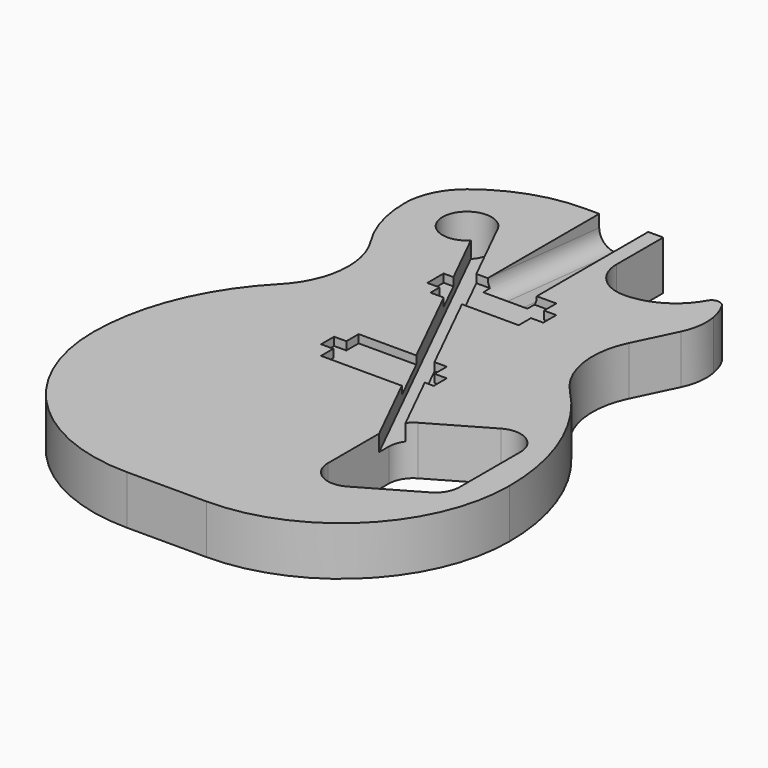
from build123d import *

# Parameters (mm, degrees)
F2_DEPTH  = 38.1
F4_R      = 19.05
F5_DEPTH  = 38.101
F11_DEPTH = 117.475
F12_W     = 9.525
F12_H     = 6.35
F13_DEPTH = 6.35
F15_DEPTH = 12.7


# Not quite as in the source:
# - a feature of the source that left no trace in its solid (it failed there, or was rolled back) is left out


with BuildPart() as f2:
    # F1 (on Top) → F2 (new body)
    with BuildSketch(Plane.XY):
        with BuildLine():
            Line((-120.142, 381.762), (0, 381.762))
            Line((0, 381.762), (0, 444.5))
            Line((0, 444.5), (-30.734, 444.5))
            ThreePointArc((-30.734, 444.5), (-68.3812374672, 438.1220807393), (-101.8270568949, 419.700096432))
            ThreePointArc((-101.8270568949, 419.700096432), (-115.3236770577, 402.8258096141), (-120.142, 381.762))
        make_face()
        with BuildLine():
            Line((0, 444.5), (0, 381.762))
            Line((0, 381.762), (36.5448035283, 381.762))
            ThreePointArc((36.5448035283, 381.762), (32.2256329717, 389.9223670283), (30.734, 399.034))
            Line((30.734, 399.034), (30.734, 444.5))
            Line((30.734, 444.5), (0, 444.5))
        make_face()
        with BuildLine():
            Line((0, 381.762), (0, 295.402))
            Line((0, 295.402), (94.869, 295.402))
            ThreePointArc((94.869, 295.402), (96.466719449, 309.5567752573), (101.1794775617, 322.9992557201))
            Line((101.1794775617, 322.9992557201), (116.4239761752, 354.5902807248))
            ThreePointArc((116.4239761752, 354.5902807248), (120.430931673, 367.882227955), (120.142, 381.762))
            Line((120.142, 381.762), (91.175550227, 381.762))
            ThreePointArc((91.175550227, 381.762), (76.2148779155, 373.3684407202), (59.309, 370.459))
            ThreePointArc((59.309, 370.459), (46.6010649789, 373.440270055), (36.5448035283, 381.762))
            Line((36.5448035283, 381.762), (0, 381.762))
        make_face()
        with BuildLine():
            ThreePointArc((103.5459630182, 396.5232874828), (98.0699350262, 388.5483304334), (91.175550227, 381.762))
            Line((91.175550227, 381.762), (120.142, 381.762))
            ThreePointArc((120.142, 381.762), (118.0226976621, 389.4849479409), (114.552023257, 396.7022733785))
            ThreePointArc((114.552023257, 396.7022733785), (112.2345927331, 398.9686730826), (109.1004928586, 399.796))
            ThreePointArc((109.1004928586, 399.796), (105.8770068198, 398.9169814255), (103.5459630182, 396.5232874828))
        make_face()
        with BuildLine():
            Line((94.869, 295.402), (0, 295.402))
            Line((0, 295.402), (0, 0))
            Line((0, 0), (30.906359714, 0))
            ThreePointArc((30.906359714, 0), (123.5505287221, 38.3744712779), (161.925, 131.018640286))
            ThreePointArc((161.925, 131.018640286), (149.2199863218, 195.80132063), (112.9871937272, 250.9864434976))
            ThreePointArc((112.9871937272, 250.9864434976), (99.5727641582, 271.4175748279), (94.869, 295.402))
        make_face()
        with BuildLine():
            Line((0, 295.402), (-94.869, 295.402))
            ThreePointArc((-94.869, 295.402), (-99.5727641582, 271.4175748279), (-112.9871937272, 250.9864434976))
            ThreePointArc((-112.9871937272, 250.9864434976), (-149.2199863218, 195.80132063), (-161.925, 131.018640286))
            ThreePointArc((-161.925, 131.018640286), (-123.5505287221, 38.3744712779), (-30.906359714, 0))
            Line((-30.906359714, 0), (0, 0))
            Line((0, 0), (0, 295.402))
        make_face()
        with BuildLine():
            ThreePointArc((-104.887559724, 329.6362744337), (-97.4250853837, 313.2370573657), (-94.869, 295.402))
            Line((-94.869, 295.402), (0, 295.402))
            Line((0, 295.402), (0, 381.762))
            Line((0, 381.762), (-120.142, 381.762))
            ThreePointArc((-120.142, 381.762), (-116.2500581541, 354.6060190108), (-104.887559724, 329.6362744337))
        make_face()
    extrude(amount=F2_DEPTH)

    # F4 (on face) → F5 (cut, through all)
    with BuildSketch(Plane.XY.offset(38.1)):
        with Locations((-71.6915, 381.762)):
            Circle(F4_R)
        with BuildLine():
            Line((139.2962010965, 110.8024764079), (139.2962010965, 170.1017752607))
            ThreePointArc((139.2962010965, 170.1017752607), (129.7712010965, 186.5995592028), (110.7212010965, 186.5995592028))
            Line((110.7212010965, 186.5995592028), (66.675, 161.169473143))
            ThreePointArc((66.675, 161.169473143), (59.7022160579, 154.1966892009), (57.15, 144.6716892009))
            Line((57.15, 144.6716892009), (57.15, 108.5037669007))
            Line((57.15, 108.5037669007), (69.5417475728, 132.0304736397))
            ThreePointArc((69.5417475728, 132.0304736397), (65.9030700587, 154.5765309479), (88.5733379566, 151.8154392009))
            Line((88.5733379566, 151.8154392009), (107.8728631399, 162.9580252607))
            ThreePointArc((107.8728631399, 162.9580252607), (116.5483239896, 183.9024405039), (134.5337010965, 170.1017752607))
            ThreePointArc((134.5337010965, 170.1017752607), (130.3489892327, 159.9989871245), (120.2462010965, 155.8142752607))
            Line((120.2462010965, 155.8142752607), (120.2462010965, 125.0899764079))
            ThreePointArc((120.2462010965, 125.0899764079), (130.3489892327, 120.9052645441), (134.5337010965, 110.8024764079))
            ThreePointArc((134.5337010965, 110.8024764079), (125.4430565732, 97.4936316269), (109.7392514861, 101.1207066247))
            Line((109.7392514861, 101.1207066247), (90.3263274862, 83.23240717))
            ThreePointArc((90.3263274862, 83.23240717), (85.8817697832, 74.8654407377), (77.1799912803, 71.1185391723))
            Line((77.1799912803, 71.1185391723), (72.3922577123, 66.7068177967))
            ThreePointArc((72.3922577123, 66.7068177967), (79.2572186381, 66.5693077763), (85.725, 68.874606406))
            Line((85.725, 68.874606406), (129.7712010965, 94.3046924658))
            ThreePointArc((129.7712010965, 94.3046924658), (136.7439850386, 101.2774764079), (139.2962010965, 110.8024764079))
        make_face()
        with BuildLine():
            Line((69.5417475728, 132.0304736397), (57.15, 108.5037669007))
            Line((57.15, 108.5037669007), (57.15, 85.3723903481))
            ThreePointArc((57.15, 85.3723903481), (61.4446621425, 73.3232200567), (72.3922577123, 66.7068177967))
            Line((72.3922577123, 66.7068177967), (77.1799912803, 71.1185391723))
            ThreePointArc((77.1799912803, 71.1185391723), (85.8817697832, 74.8654407377), (90.3263274862, 83.23240717))
            Line((90.3263274862, 83.23240717), (109.7392514861, 101.1207066247))
            ThreePointArc((109.7392514861, 101.1207066247), (125.4430565732, 97.4936316269), (134.5337010965, 110.8024764079))
            ThreePointArc((134.5337010965, 110.8024764079), (130.3489892327, 120.9052645441), (120.2462010965, 125.0899764079))
            Line((120.2462010965, 125.0899764079), (120.2462010965, 155.8142752607))
            ThreePointArc((120.2462010965, 155.8142752607), (130.3489892327, 159.9989871245), (134.5337010965, 170.1017752607))
            ThreePointArc((134.5337010965, 170.1017752607), (116.5483239896, 183.9024405039), (107.8728631399, 162.9580252607))
            Line((107.8728631399, 162.9580252607), (88.5733379566, 151.8154392009))
            ThreePointArc((88.5733379566, 151.8154392009), (65.9030700587, 154.5765309479), (69.5417475728, 132.0304736397))
        make_face()
    extrude(amount=-F5_DEPTH, mode=Mode.SUBTRACT)

    # F10 (on face) → F11 (cut)
    with BuildSketch(Plane(origin=(0, 441.123523107, -38.5933074865), x_dir=(-1, 0, 0), z_dir=(0, 0.9961946981, -0.0871557427))):
        with BuildLine():
            Line((19.05, 76.6957456486), (-19.05, 76.6957456486))
            Line((-19.05, 76.6957456486), (-19.05, 67.1707456486))
            ThreePointArc((-19.05, 67.1707456486), (-15.3302561211, 58.1904895276), (-6.35, 54.4707456486))
            Line((-6.35, 54.4707456486), (0, 54.4707456486))
            Line((0, 54.4707456486), (6.35, 54.4707456486))
            ThreePointArc((6.35, 54.4707456486), (15.3302561211, 58.1904895276), (19.05, 67.1707456486))
            Line((19.05, 67.1707456486), (19.05, 76.6957456486))
        make_face()
    extrude(amount=-F11_DEPTH, mode=Mode.SUBTRACT)

    # F12 (on face) → F13 (cut)
    with BuildSketch(Plane.XY.offset(38.1)):
        Polygon((-34.29, 299.5168), (0, 299.5168), (0, 317.8302), (-34.29, 317.8302), (-34.29, 311.4802), (-34.29, 308.3052), align=None)
        Polygon((0, 317.8302), (0, 299.5168), (34.29, 299.5168), (34.29, 311.4802), (34.29, 317.8302), align=None)
        Polygon((0, 229.6668), (-34.29, 229.6668), (-34.29, 217.7034), (-34.29, 211.3534), (0, 211.3534), align=None)
        Polygon((34.29, 229.6668), (0, 229.6668), (0, 211.3534), (34.29, 211.3534), (34.29, 217.7034), align=None)
        with Locations((-39.0525, 214.5284)):
            Rectangle(F12_W, F12_H)
        Polygon((34.29, 211.3534), (0, 211.3534), (0, 193.04), (34.29, 193.04), (34.29, 205.0034), align=None)
        Polygon((0, 193.04), (0, 211.3534), (-34.29, 211.3534), (-34.29, 205.0034), (-34.29, 193.04), align=None)
        with Locations((-39.0525, 208.1784)):
            Rectangle(F12_W, F12_H)
        with Locations((39.0525, 214.5284)):
            Rectangle(F12_W, F12_H)
        Polygon((0, 336.1436), (0, 317.8302), (34.29, 317.8302), (34.29, 324.1802), (34.29, 336.1436), align=None)
        Polygon((-34.29, 317.8302), (0, 317.8302), (0, 336.1436), (-34.29, 336.1436), (-34.29, 324.1802), align=None)
        with Locations((39.0525, 208.1784)):
            Rectangle(F12_W, F12_H)
        Polygon((-43.815, 308.3052), (-34.29, 308.3052), (-34.29, 311.4802), (-34.29, 317.8302), (-43.815, 317.8302), (-43.815, 311.4802), align=None)
        with Locations((39.0525, 314.6552)):
            Rectangle(F12_W, F12_H)
        with Locations((39.0525, 321.0052)):
            Rectangle(F12_W, F12_H)
        with Locations((-39.0525, 321.0052)):
            Rectangle(F12_W, F12_H)
    extrude(amount=-F13_DEPTH, mode=Mode.SUBTRACT)

    # F14 (on face) → F15 (cut)
    with BuildSketch(Plane.XY.offset(38.1)):
        with BuildLine():
            Line((-54.0675192427, 388.9937219434), (-58.0760770823, 368.4382333114))
            Line((-58.0760770823, 368.4382333114), (57.15, 135.255))
            Line((57.15, 135.255), (57.15, 144.6716892009))
            ThreePointArc((57.15, 144.6716892009), (58.1362792436, 150.7218538627), (60.9929913317, 156.1455458918))
            Line((60.9929913317, 156.1455458918), (-54.0675192427, 388.9937219434))
        make_face()
    extrude(amount=-F15_DEPTH, mode=Mode.SUBTRACT)


solid = f2.part
